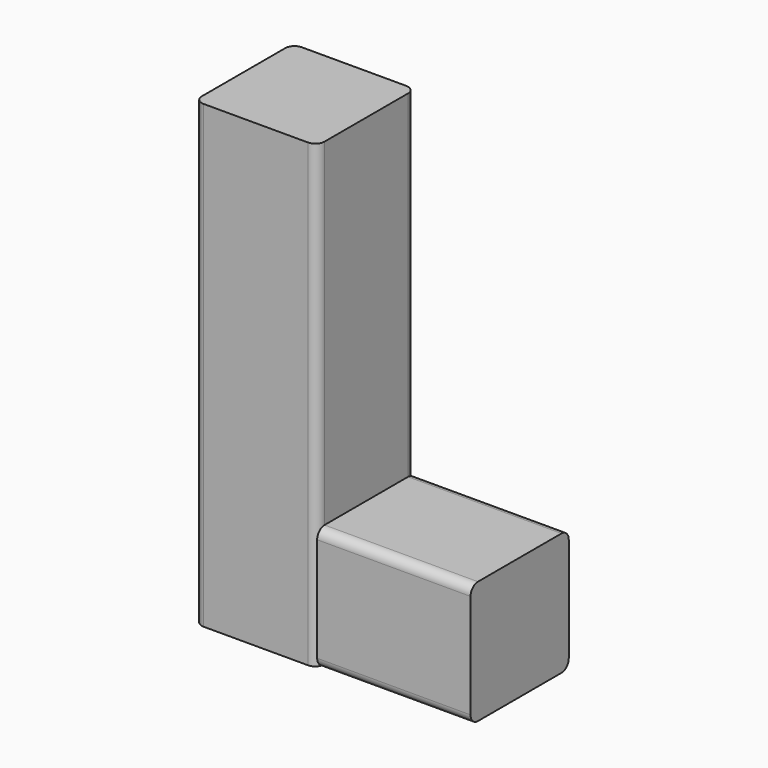
from build123d import *

# Parameters (mm, degrees)
F0_W        = 80
F0_H        = 80
F1_DEPTH    = 300
F2_R        = 6
F3_W        = 80
F3_H        = 80
F4_DEPTH    = 100
F5_T1_DEPTH = 115


# Not quite as in the source:
# - a fillet or chamfer that OpenCascade refuses, or shapes differently, is made with other operations: its cross-section is extruded or revolved along the edge and cut away or added


with BuildPart() as f1:
    # F0 (on Top) → F1 (new body)
    with BuildSketch(Plane.XY):
        with Locations((-40, 40)):
            Rectangle(F0_W, F0_H)
    extrude(amount=F1_DEPTH)

    # F2
    f2_edges = [f1.edges().sort_by_distance(p)[0] for p in [
        (-80, 80, 150),
        (-80, 0, 150),
        (0, 0, 150),
        (0, 80, 150),
    ]]
    fillet(f2_edges, radius=F2_R)

    # F3 (on Right) → F4 (join)
    with BuildSketch(Plane.YZ):
        with Locations((40, 40)):
            Rectangle(F3_W, F3_H)
    extrude(amount=F4_DEPTH)

    # F5: fillet of radius 6 on 4 edges, made by hand

    # F5_s2 → F5_t1 (cut)
    with BuildSketch(Plane.YZ):
        with BuildLine():
            ThreePointArc((0, 74), (1.7573593129, 78.2426406871), (6, 80))
            Line((6, 80), (0, 80))
            Line((0, 80), (0, 74))
        make_face()
        with BuildLine():
            ThreePointArc((80, 74), (78.2426406871, 78.2426406871), (74, 80))
            Line((74, 80), (80, 80))
            Line((80, 80), (80, 74))
        make_face()
        with BuildLine():
            ThreePointArc((6, 0), (1.7573593129, 1.7573593129), (0, 6))
            Line((0, 6), (0, 0))
            Line((0, 0), (6, 0))
        make_face()
        with BuildLine():
            ThreePointArc((74, 0), (78.2426406871, 1.7573593129), (80, 6))
            Line((80, 6), (80, 0))
            Line((80, 0), (74, 0))
        make_face()
    extrude(amount=F5_T1_DEPTH, mode=Mode.SUBTRACT)


solid = f1.part
